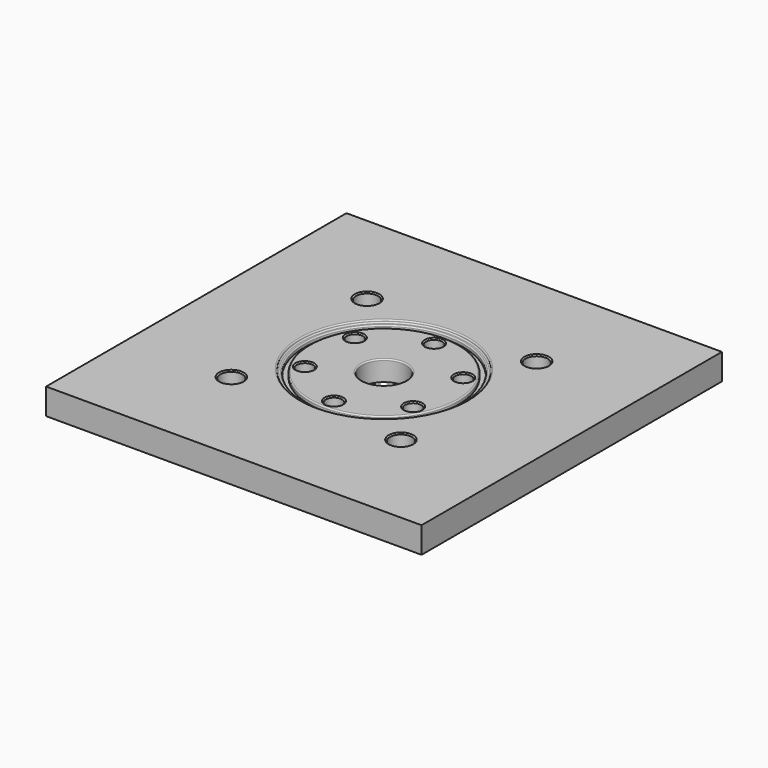
from build123d import *

# Parameters (mm, degrees)
F1_DEPTH  = 15.875
F2_R      = 6.746875
F3_DEPTH  = 25.4
F4_R      = 50.927
F4_R_2    = 13.49375
F5_DEPTH  = 1.5875
F6_DEPTH  = 25.4
F7_R      = 50.927
F7_R_2    = 13.49375
F8_DEPTH  = 1.5875
F9_R      = 4.953
F10_DEPTH = 25.4
F9_R_2    = 48.4886
F9_R_3    = 45.4914
F11_DEPTH = 4.1275
F12_R     = 48.4886
F12_R_2   = 45.4914
F13_DEPTH = 2.54
F14_R     = 0.762
F15_SIZE  = 0.762


# Not quite as in the source:
# - a feature names something its author has since deleted; it is built from what else it names


with BuildPart() as f1:
    # F0 (on Top) → F1 (new body)
    with BuildSketch(Plane.XY):
        with BuildLine():
            ThreePointArc((58.9450638246, 74.8200638246), (77.4288162629, 55.4737858103), (89.8025612107, 31.75))
            Line((89.8025612107, 31.75), (114.3, 74.1808086384))
            Line((114.3, 74.1808086384), (114.3, 114.3))
            Line((114.3, 114.3), (98.425, 114.3))
            Line((98.425, 114.3), (58.9450638246, 74.8200638246))
        make_face()
        with BuildLine():
            ThreePointArc((-89.8025612107, 31.75), (-77.4288162629, 55.4737858103), (-58.9450638246, 74.8200638246))
            Line((-58.9450638246, 74.8200638246), (-98.425, 114.3))
            Line((-98.425, 114.3), (-114.3, 114.3))
            Line((-114.3, 114.3), (-114.3, 74.1808086384))
            Line((-114.3, 74.1808086384), (-89.8025612107, 31.75))
        make_face()
        with BuildLine():
            Line((-98.425, -114.3), (-58.9450638246, -74.8200638246))
            ThreePointArc((-58.9450638246, -74.8200638246), (-77.4288162629, -55.4737858103), (-89.8025612107, -31.75))
            Line((-89.8025612107, -31.75), (-114.3, -74.1808086384))
            Line((-114.3, -74.1808086384), (-114.3, -114.3))
            Line((-114.3, -114.3), (-98.425, -114.3))
        make_face()
        with BuildLine():
            Line((114.3, -74.1808086384), (89.8025612107, -31.75))
            ThreePointArc((89.8025612107, -31.75), (77.4288162629, -55.4737858103), (58.9450638246, -74.8200638246))
            Line((58.9450638246, -74.8200638246), (98.425, -114.3))
            Line((98.425, -114.3), (114.3, -114.3))
            Line((114.3, -114.3), (114.3, -74.1808086384))
        make_face()
        with BuildLine():
            ThreePointArc((89.8025612107, -31.75), (93.878262807, -16.1069634736), (95.25, 0))
            ThreePointArc((95.25, 0), (93.878262807, 16.1069634736), (89.8025612107, 31.75))
            ThreePointArc((89.8025612107, 31.75), (77.4288162629, 55.4737858103), (58.9450638246, 74.8200638246))
            ThreePointArc((58.9450638246, 74.8200638246), (0, 95.25), (-58.9450638246, 74.8200638246))
            ThreePointArc((-58.9450638246, 74.8200638246), (-77.4288162629, 55.4737858103), (-89.8025612107, 31.75))
            ThreePointArc((-89.8025612107, 31.75), (-95.25, 0), (-89.8025612107, -31.75))
            ThreePointArc((-89.8025612107, -31.75), (-77.4288162629, -55.4737858103), (-58.9450638246, -74.8200638246))
            ThreePointArc((-58.9450638246, -74.8200638246), (0, -95.25), (58.9450638246, -74.8200638246))
            ThreePointArc((58.9450638246, -74.8200638246), (77.4288162629, -55.4737858103), (89.8025612107, -31.75))
        make_face()
        with BuildLine():
            ThreePointArc((-58.9450638246, 74.8200638246), (0, 95.25), (58.9450638246, 74.8200638246))
            Line((58.9450638246, 74.8200638246), (98.425, 114.3))
            Line((98.425, 114.3), (-98.425, 114.3))
            Line((-98.425, 114.3), (-58.9450638246, 74.8200638246))
        make_face()
        with BuildLine():
            ThreePointArc((89.8025612107, 31.75), (93.878262807, 16.1069634736), (95.25, 0))
            ThreePointArc((95.25, 0), (93.878262807, -16.1069634736), (89.8025612107, -31.75))
            Line((89.8025612107, -31.75), (114.3, -74.1808086384))
            Line((114.3, -74.1808086384), (114.3, 74.1808086384))
            Line((114.3, 74.1808086384), (89.8025612107, 31.75))
        make_face()
        with BuildLine():
            Line((98.425, -114.3), (58.9450638246, -74.8200638246))
            ThreePointArc((58.9450638246, -74.8200638246), (0, -95.25), (-58.9450638246, -74.8200638246))
            Line((-58.9450638246, -74.8200638246), (-98.425, -114.3))
            Line((-98.425, -114.3), (98.425, -114.3))
        make_face()
        with BuildLine():
            ThreePointArc((-89.8025612107, -31.75), (-95.25, 0), (-89.8025612107, 31.75))
            Line((-89.8025612107, 31.75), (-114.3, 74.1808086384))
            Line((-114.3, 74.1808086384), (-114.3, -74.1808086384))
            Line((-114.3, -74.1808086384), (-89.8025612107, -31.75))
        make_face()
    extrude(amount=F1_DEPTH)

    # F2 (on face) → F3 (cut)
    with BuildSketch(Plane.XY.offset(15.875)):
        with Locations((51.6364726961, 51.6364726961)):
            Circle(F2_R)
        with Locations((-51.6364726961, 51.6364726961)):
            Circle(F2_R)
        with Locations((-51.6364726961, -51.6364726961)):
            Circle(F2_R)
        with Locations((51.6364726961, -51.6364726961)):
            Circle(F2_R)
    extrude(amount=-F3_DEPTH, mode=Mode.SUBTRACT)

    # F4 (on face) → F5 (cut)
    with BuildSketch(Plane.XY.offset(15.875)):
        Circle(F4_R)
        Circle(F4_R_2, mode=Mode.SUBTRACT)
    extrude(amount=-F5_DEPTH, mode=Mode.SUBTRACT)

    # F4 (on face) → F6 (cut)
    with BuildSketch(Plane.XY.offset(15.875)):
        Circle(F4_R_2)
    extrude(amount=-F6_DEPTH, mode=Mode.SUBTRACT)

    # F7 (on face) → F8 (cut)
    with BuildSketch(Plane(origin=(0, 0, 0), x_dir=(1, 0, 0), z_dir=(0, 0, -1))):
        Circle(F7_R)
        Circle(F7_R_2, mode=Mode.SUBTRACT)
    extrude(amount=-F8_DEPTH, mode=Mode.SUBTRACT)

    # F9 (on face) → F10 (cut)
    with BuildSketch(Plane.XY.offset(15.875)):
        with Locations((0, 38.1)):
            Circle(F9_R)
        with Locations((32.9955678842, 19.05)):
            Circle(F9_R)
        with Locations((-32.9955678842, 19.05)):
            Circle(F9_R)
        with Locations((-32.9955678842, -19.05)):
            Circle(F9_R)
        with Locations((0, -38.1)):
            Circle(F9_R)
        with Locations((32.9955678842, -19.05)):
            Circle(F9_R)
    extrude(amount=-F10_DEPTH, mode=Mode.SUBTRACT)

    # F9 (on face) → F11 (cut)
    with BuildSketch(Plane.XY.offset(15.875)):
        Circle(F9_R_2)
        Circle(F9_R_3, mode=Mode.SUBTRACT)
    extrude(amount=-F11_DEPTH, mode=Mode.SUBTRACT)

    # F12 (on face) → F13 (cut)
    with BuildSketch(Plane(origin=(0, 0, 1.5875), x_dir=(1, 0, 0), z_dir=(0, 0, -1))):
        Circle(F12_R)
        Circle(F12_R_2, mode=Mode.SUBTRACT)
    extrude(amount=-F13_DEPTH, mode=Mode.SUBTRACT)

    # F14
    f14_edges = [f1.edges().sort_by_distance(p)[0] for p in [
        (-50.927, 0, 0),
        (-50.927, 0, 1.5875),
        (-48.4886, 0, 1.5875),
        (-45.4914, 0, 1.5875),
        (-13.49375, 0, 1.5875),
        (-13.49375, 0, 14.2875),
        (-48.4886, 0, 14.2875),
        (-50.927, 0, 14.2875),
        (-50.927, 0, 15.875),
        (-45.4914, 0, 14.2875),
    ]]
    fillet(f14_edges, radius=F14_R)

    # F15
    f15_edges = [f1.edges().sort_by_distance(p)[0] for p in [
        (44.889598, 51.636473, 15.875),
        (44.889598, 51.636473, 0),
        (44.889598, -51.636473, 15.875),
        (44.889598, -51.636473, 0),
        (-58.383348, 51.636473, 0),
        (-58.383348, 51.636473, 15.875),
        (-58.383348, -51.636473, 0),
        (-58.383348, -51.636473, 15.875),
        (-4.953, 38.1, 1.5875),
        (-4.953, 38.1, 14.2875),
        (28.042568, 19.05, 1.5875),
        (28.042568, 19.05, 14.2875),
        (28.042568, -19.05, 1.5875),
        (28.042568, -19.05, 14.2875),
        (-4.953, -38.1, 1.5875),
        (-4.953, -38.1, 14.2875),
        (-37.948568, -19.05, 1.5875),
        (-37.948568, -19.05, 14.2875),
        (-37.948568, 19.05, 14.2875),
        (-37.948568, 19.05, 1.5875),
    ]]
    chamfer(f15_edges, length=F15_SIZE)


solid = f1.part
